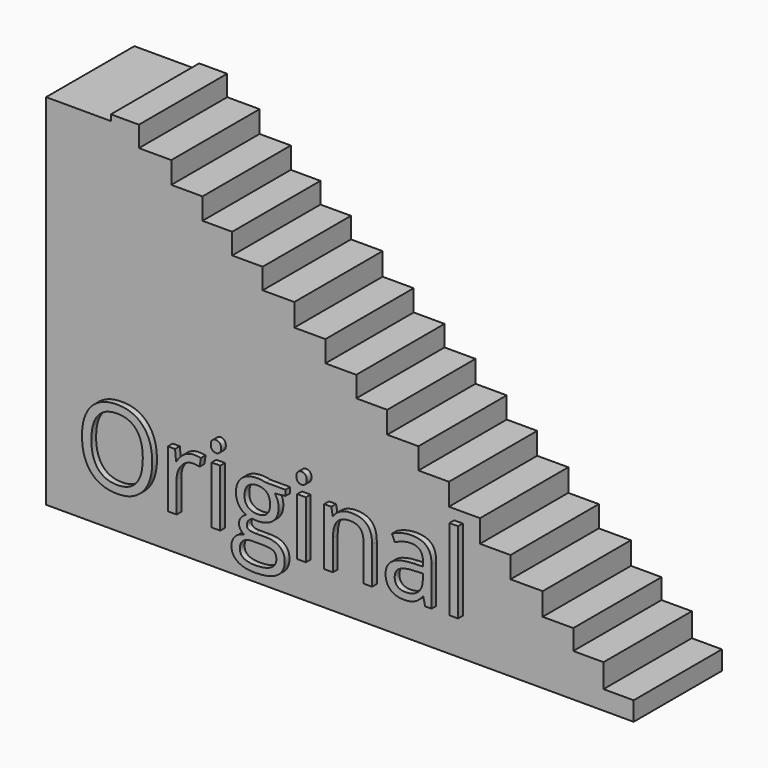
from build123d import *

# Parameters (mm, degrees)
F1_DEPTH     = 93
F2_TEXT_SIZE = 90.1304909752
F3_DEPTH     = 5


# Not quite as in the source:
# - Text() gives the source's letters only with a copy of the font that has no kerning and outlines rounded to 1/6400 em; it was checked with that copy


with BuildPart() as f1:
    # F0 (on Front) → F1 (new body)
    with BuildSketch(Plane.XZ):
        Polygon((-495.2547848225, 0), (0, 0), (0, 16), (-25.4, 16), (-25.4, 36), (-50.9, 36), (-50.9, 53), (-76.7, 53), (-76.7, 72), (-103.8, 72), (-103.8, 90), (-129.5, 90), (-129.5, 109), (-155.7, 109), (-155.7, 127.5), (-181.4, 127.5), (-181.4, 145.5), (-207.7, 145.5), (-207.7, 164), (-233.8, 164), (-233.8, 181.5), (-259.8, 181.5), (-259.8, 199.5), (-286, 199.5), (-286, 218.5), (-312.7, 218.5), (-312.7, 236), (-338.4, 236), (-338.4, 253.6), (-363.4, 253.6), (-363.4, 271.7), (-389.7, 271.7), (-389.7, 290.1), (-417, 290.1), (-417, 307.5), (-440.6500756741, 307.5), (-440.6500756741, 302.5), (-495.2547848225, 302.5), align=None)
    extrude(amount=F1_DEPTH)

    # F2 (on face) → F3 (join)
    with BuildSketch(Plane.XZ.offset(93)):
        with Locations((-466.4991348982, 31.862705946)):
            Text('Original', F2_TEXT_SIZE, font='Open Sans', text_align=(TextAlign.LEFT, TextAlign.BOTTOM))
    extrude(amount=F3_DEPTH)


solid = f1.part
